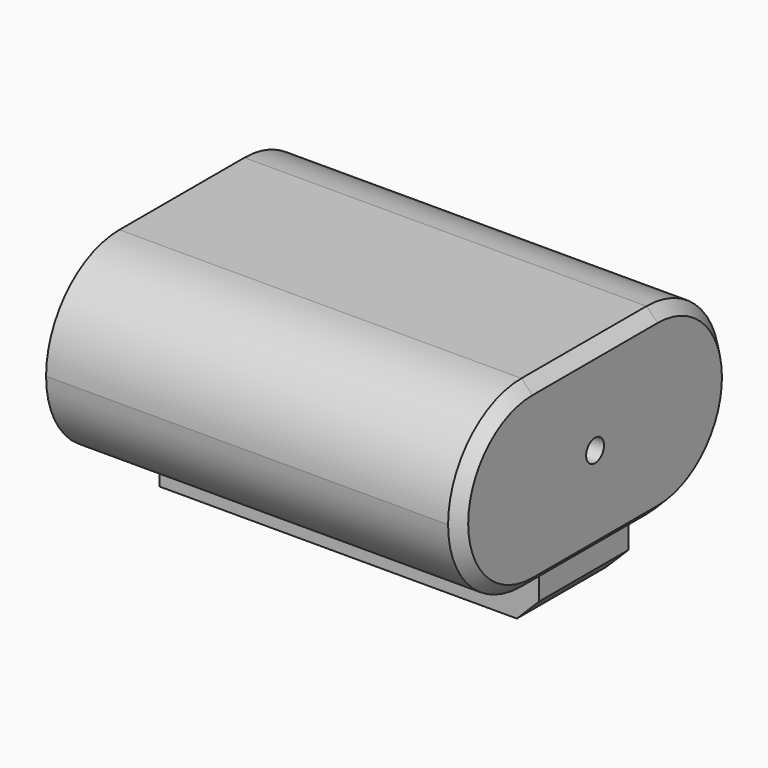
from build123d import *

# Parameters (mm, degrees)
F1_DEPTH    = 35
F2_T        = 2
F3_T1_DEPTH = 14
F3_T4_ANGLE = 180
F3_T6_ANGLE = 180
F4_R        = 1
F5_DEPTH    = 3
F6_W        = 1
F6_H        = 10
F6_W_2      = 33
F7_DEPTH    = 4
F8_SIZE     = 2


# Not quite as in the source:
# - a fillet or chamfer that OpenCascade refuses, or shapes differently, is made with other operations: its cross-section is extruded or revolved along the edge and cut away or added


with BuildPart() as f1:
    # F0 (on Right) → F1 (new body)
    with BuildSketch(Plane.YZ):
        with BuildLine():
            ThreePointArc((-8.5429217076, 0.448732347), (-6.726983751, -3.9353296963), (-2.3429217076, -5.751267653))
            Line((-2.3429217076, -5.751267653), (11.6570782924, -5.751267653))
            ThreePointArc((11.6570782924, -5.751267653), (16.0411403357, -3.9353296963), (17.8570782924, 0.448732347))
            ThreePointArc((17.8570782924, 0.448732347), (16.0411403357, 4.8327943904), (11.6570782924, 6.648732347))
            Line((11.6570782924, 6.648732347), (-2.3429217076, 6.648732347))
            ThreePointArc((-2.3429217076, 6.648732347), (-6.726983751, 4.8327943904), (-8.5429217076, 0.448732347))
        make_face()
    extrude(amount=F1_DEPTH)

    # F2
    f2_openings = [f1.faces().sort_by_distance(p)[0] for p in [
        (0, 4.657078, 0.448732),
    ]]
    offset(amount=F2_T, openings=f2_openings, kind=Kind.INTERSECTION)

    # F3: chamfer of 1 on 4 edges, made by hand

    # F3_s2 → F3_t1 (cut)
    with BuildSketch(Plane.XZ.offset(-11.6570782924)):
        Polygon((37, -6.751267653), (36, -7.751267653), (37, -7.751267653), align=None)
        Polygon((37, 7.648732347), (36, 8.648732347), (37, 8.648732347), align=None)
    extrude(amount=F3_T1_DEPTH, mode=Mode.SUBTRACT)

    # F3_s3 → F3_t4 (revolve, cut)
    with BuildSketch(Plane.XZ.offset(2.3429217076)):
        Polygon((36, -7.751267653), (37, -6.751267653), (37, -7.751267653), align=None)
    revolve(axis=Axis((37, -2.3429217076, 0.448732347), (-1, 0, 0)), revolution_arc=F3_T4_ANGLE, mode=Mode.SUBTRACT)

    # F3_s5 → F3_t6 (revolve, cut)
    with BuildSketch(Plane.XZ.offset(-11.6570782924)):
        Polygon((37, 7.648732347), (36, 8.648732347), (37, 8.648732347), align=None)
    revolve(axis=Axis((37, 11.6570782924, 0.448732347), (-1, 0, 0)), revolution_arc=F3_T6_ANGLE, mode=Mode.SUBTRACT)

    # F4 (on face) → F5 (cut)
    with BuildSketch(Plane.YZ.offset(37)):
        with Locations((4.6570782924, 0.448732347)):
            Circle(F4_R)
    extrude(amount=-F5_DEPTH, mode=Mode.SUBTRACT)

    # F6 (on face) → F7 (join)
    with BuildSketch(Plane(origin=(0, 0, -7.751267653), x_dir=(1, 0, 0), z_dir=(0, 0, -1))):
        with Locations((35.5, -4.6570782924)):
            Rectangle(F6_W, F6_H)
        with Locations((18.5, -4.6570782924)):
            Rectangle(F6_W_2, F6_H)
    extrude(amount=F7_DEPTH)

    # F8
    f8_edges = [f1.edges().sort_by_distance(p)[0] for p in [
        (36, 4.657078, -11.751268),
    ]]
    chamfer(f8_edges, length=F8_SIZE)


solid = f1.part
